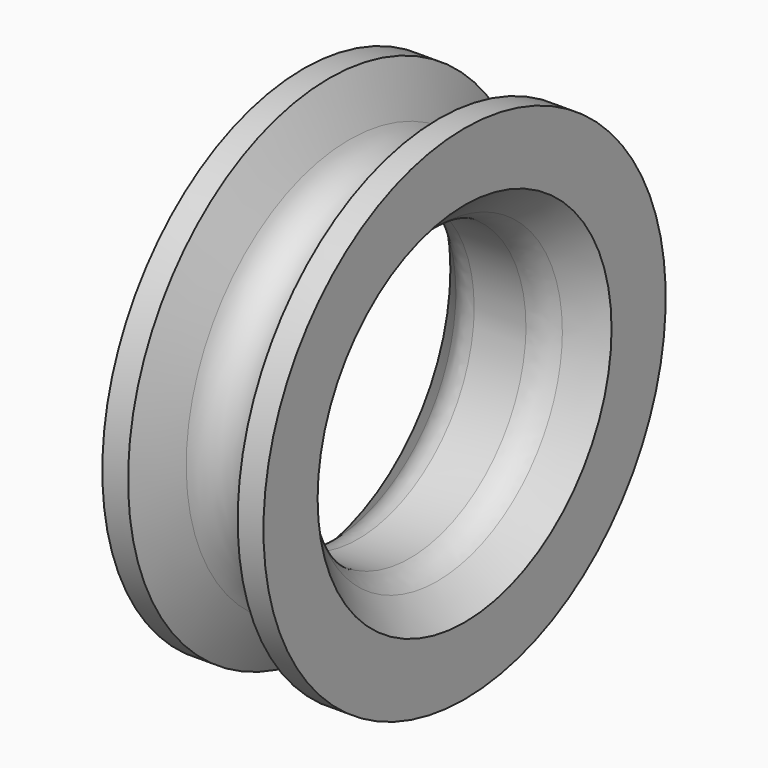
from build123d import *

# Parameters (mm, degrees)
F1_R     = 5
F1_R_2   = 4.5
F3_DEPTH = 2.5
F5_SIZE  = 1.2
F6_R     = 1.2


with BuildPart() as f3:
    # F1 (on Right) → F3 (new body, symmetric)
    with BuildSketch(Plane.YZ):
        Circle(F1_R)
        Circle(F1_R_2, mode=Mode.SUBTRACT)
    extrude(amount=F3_DEPTH, both=True)

    # F2 (on Front) → F4 (revolve)
    with BuildSketch(Plane.XZ):
        with BuildLine():
            Line((-2.5, 7.8), (-2.5, 5))
            Line((-2.5, 5), (0, 5))
            Line((0, 5), (2.5, 5))
            Line((2.5, 5), (2.5, 7.8))
            Line((2.5, 7.8), (1.7, 7.8))
            Line((1.7, 7.8), (1.0748301944, 6.3271922345))
            ThreePointArc((1.0748301944, 6.3271922345), (0, 5.6157776481), (-1.0748301944, 6.3271922345))
            Line((-1.0748301944, 6.3271922345), (-1.7, 7.8))
            Line((-1.7, 7.8), (-2.5, 7.8))
        make_face()
    revolve(axis=Axis((0, 0, 0), (1, 0, 0)))

    # F5
    f5_edges = [f3.edges().sort_by_distance(p)[0] for p in [
        (-2.5, -4.5, 0),
        (2.5, -4.5, 0),
    ]]
    chamfer(f5_edges, length=F5_SIZE)

    # F6
    f6_edges = [f3.edges().sort_by_distance(p)[0] for p in [
        (1.3, -4.5, 0),
        (-1.3, -4.5, 0),
    ]]
    fillet(f6_edges, radius=F6_R)


solid = f3.part
